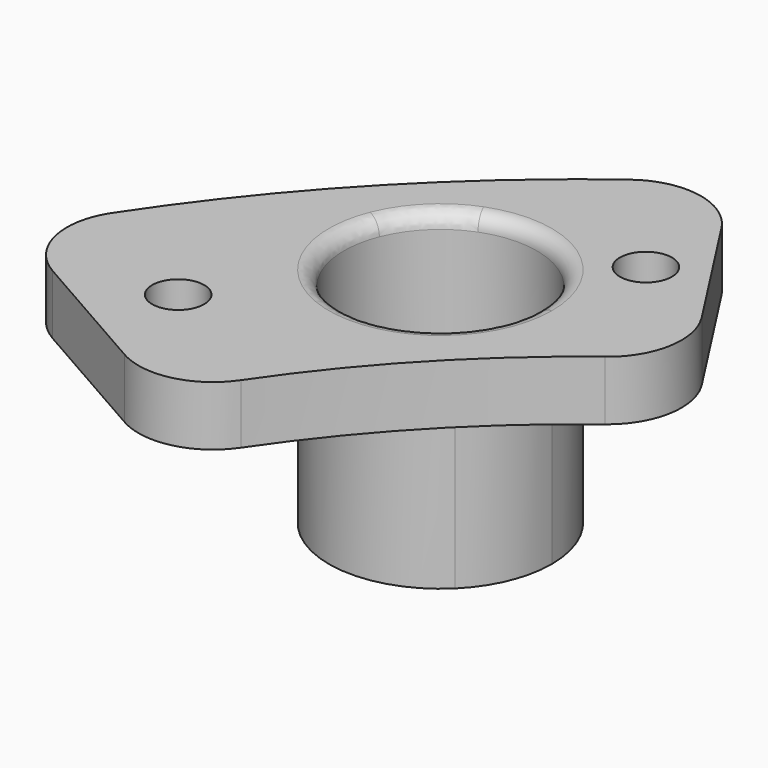
from build123d import *

# Parameters (mm, degrees)
F0_R     = 1.75
F1_DEPTH = 4
F2_DEPTH = 15
F3_R     = 5
F4_R     = 1


# Not quite as in the source:
# - a feature names something its author has since deleted; it is built from what else it names


with BuildPart() as f1:
    # F0 (on Top) → F1 (new body)
    with BuildSketch(Plane.XY):
        with BuildLine():
            Line((-33.9130103109, 52.4991212465), (-41.2382205381, 63.8389314357))
            ThreePointArc((-41.2382205381, 63.8389314357), (-44.9500240756, 61.2820963709), (-48.5037329382, 58.5097247563))
            ThreePointArc((-48.5037329382, 58.5097247563), (-49.20563764, 57.9206804556), (-49.9003894351, 57.3232163633))
            ThreePointArc((-49.9003894351, 57.3232163633), (-44.1059919264, 55.4322284704), (-41.6292667465, 49.8629637))
            ThreePointArc((-41.6292667465, 49.8629637), (-42.2108537269, 46.9671803363), (-43.8654164238, 44.5205036131))
            ThreePointArc((-43.8654164238, 44.5205036131), (-39.0932922784, 48.7643773551), (-33.9130103109, 52.4991212465))
        make_face()
        with Locations((-40.8724684836, 56.828173647)):
            Circle(F0_R, mode=Mode.SUBTRACT)
        with BuildLine():
            ThreePointArc((-49.4610434567, 59.6645219554), (-51.9749220296, 57.4878898553), (-54.3931164452, 55.2054244018))
            ThreePointArc((-54.3931164452, 55.2054244018), (-52.3271541158, 56.6470271117), (-49.9003894351, 57.3232163633))
            ThreePointArc((-49.9003894351, 57.3232163633), (-49.20563764, 57.9206804556), (-48.5037329382, 58.5097247563))
            Line((-48.5037329382, 58.5097247563), (-49.4610434568, 59.6645219554))
        make_face()
        with BuildLine():
            Line((-69.4199358602, 39.5800459158), (-67.3257807989, 38.3860552782))
            ThreePointArc((-67.3257807989, 38.3860552782), (-61.4377349925, 47.2403928751), (-54.3931164452, 55.2054244018))
            ThreePointArc((-54.3931164452, 55.2054244018), (-51.9749220296, 57.4878898553), (-49.4610434567, 59.6645219554))
            Line((-49.4610434568, 59.6645219554), (-50.9995194055, 61.5203750796))
            ThreePointArc((-50.9995194055, 61.5203750796), (-61.2009461738, 51.382406687), (-69.4199358602, 39.5800459158))
        make_face()
        with BuildLine():
            ThreePointArc((-49.4610434567, 59.6645219554), (-45.8371956034, 62.4916114308), (-42.0521327855, 65.0989103456))
            Line((-42.0521327855, 65.0989103456), (-43.360156037, 67.123799043))
            ThreePointArc((-43.360156037, 67.123799043), (-47.2629524833, 64.4354006125), (-50.9995194055, 61.5203750796))
            Line((-50.9995194055, 61.5203750796), (-49.4610434568, 59.6645219554))
        make_face()
        with BuildLine():
            Line((-41.2382205381, 63.8389314357), (-42.0521327855, 65.0989103456))
            ThreePointArc((-42.0521327855, 65.0989103456), (-45.8371956034, 62.4916114308), (-49.4610434567, 59.6645219554))
            Line((-49.4610434568, 59.6645219554), (-48.5037329382, 58.5097247563))
            ThreePointArc((-48.5037329382, 58.5097247563), (-44.9500240756, 61.2820963709), (-41.2382205381, 63.8389314357))
        make_face()
        with BuildLine():
            ThreePointArc((-54.3931164452, 55.2054244018), (-61.4377349925, 47.2403928751), (-67.3257807989, 38.3860552782))
            Line((-67.3257807989, 38.3860552782), (-66.0227011705, 37.6430993696))
            ThreePointArc((-66.0227011705, 37.6430993696), (-61.6490099795, 44.4454673566), (-56.577269857, 50.7445813415))
            ThreePointArc((-56.577269857, 50.7445813415), (-55.8651839567, 53.1610569882), (-54.3931164452, 55.2054244018))
        make_face()
        with BuildLine():
            ThreePointArc((-49.9003894351, 57.3232163633), (-52.3271541158, 56.6470271117), (-54.3931164452, 55.2054244018))
            ThreePointArc((-54.3931164452, 55.2054244018), (-55.8651839567, 53.1610569882), (-56.577269857, 50.7445813415))
            ThreePointArc((-56.577269857, 50.7445813415), (-55.8760464089, 51.5157008854), (-55.1643138946, 52.277131449))
            ThreePointArc((-55.1643138946, 52.277131449), (-53.6912700872, 54.4930960436), (-51.453714731, 55.9331318663))
            ThreePointArc((-51.453714731, 55.9331318663), (-50.6818181556, 56.6334998781), (-49.9003894351, 57.3232163633))
        make_face()
        with BuildLine():
            ThreePointArc((-41.6292667465, 49.8629637), (-44.1059919264, 55.4322284704), (-49.9003894351, 57.3232163633))
            ThreePointArc((-49.9003894351, 57.3232163633), (-50.6818181556, 56.6334998781), (-51.453714731, 55.9331318663))
            ThreePointArc((-51.453714731, 55.9331318663), (-45.4454448113, 55.2182840406), (-42.6292667465, 49.8629637))
            ThreePointArc((-42.6292667465, 49.8629637), (-50.3585335071, 43.4802602578), (-55.1643138946, 52.277131449))
            ThreePointArc((-55.1643138946, 52.277131449), (-55.8760464089, 51.5157008854), (-56.577269857, 50.7445813415))
            ThreePointArc((-56.577269857, 50.7445813415), (-52.4273596413, 43.1270462972), (-43.8654164238, 44.5205036131))
            ThreePointArc((-43.8654164238, 44.5205036131), (-42.2108537269, 46.9671803363), (-41.6292667465, 49.8629637))
        make_face()
        with BuildLine():
            ThreePointArc((-56.577269857, 50.7445813415), (-61.6490099795, 44.4454673566), (-66.0227011705, 37.6430993696))
            Line((-66.0227011705, 37.6430993696), (-54.2949845152, 30.9564961921))
            ThreePointArc((-54.2949845152, 30.9564961921), (-49.5465604503, 38.0970910641), (-43.8654164238, 44.5205036131))
            ThreePointArc((-43.8654164238, 44.5205036131), (-52.4273596413, 43.1270462972), (-56.577269857, 50.7445813415))
        make_face()
        with Locations((-58.1049998349, 39.0359961341)):
            Circle(F0_R, mode=Mode.SUBTRACT)
        with BuildLine():
            ThreePointArc((-43.8654164238, 44.5205036131), (-49.5465604503, 38.0970910641), (-54.2949845152, 30.9564961921))
            Line((-54.2949845152, 30.9564961921), (-51.8884792508, 29.5844178737))
            ThreePointArc((-51.8884792508, 29.5844178737), (-43.387995367, 41.0503826769), (-32.4098910344, 50.1722136548))
            Line((-32.4098910344, 50.1722136548), (-33.9130103109, 52.4991212465))
            ThreePointArc((-33.9130103109, 52.4991212465), (-39.0932922784, 48.7643773551), (-43.8654164238, 44.5205036131))
        make_face()
    extrude(amount=-F1_DEPTH)

    # F0 (on Top) → F2 (join)
    with BuildSketch(Plane.XY):
        with BuildLine():
            ThreePointArc((-49.9003894351, 57.3232163633), (-52.3271541158, 56.6470271117), (-54.3931164452, 55.2054244018))
            ThreePointArc((-54.3931164452, 55.2054244018), (-55.8651839567, 53.1610569882), (-56.577269857, 50.7445813415))
            ThreePointArc((-56.577269857, 50.7445813415), (-55.8760464089, 51.5157008854), (-55.1643138946, 52.277131449))
            ThreePointArc((-55.1643138946, 52.277131449), (-53.6912700872, 54.4930960436), (-51.453714731, 55.9331318663))
            ThreePointArc((-51.453714731, 55.9331318663), (-50.6818181556, 56.6334998781), (-49.9003894351, 57.3232163633))
        make_face()
        with BuildLine():
            ThreePointArc((-41.6292667465, 49.8629637), (-44.1059919264, 55.4322284704), (-49.9003894351, 57.3232163633))
            ThreePointArc((-49.9003894351, 57.3232163633), (-50.6818181556, 56.6334998781), (-51.453714731, 55.9331318663))
            ThreePointArc((-51.453714731, 55.9331318663), (-45.4454448113, 55.2182840406), (-42.6292667465, 49.8629637))
            ThreePointArc((-42.6292667465, 49.8629637), (-50.3585335071, 43.4802602578), (-55.1643138946, 52.277131449))
            ThreePointArc((-55.1643138946, 52.277131449), (-55.8760464089, 51.5157008854), (-56.577269857, 50.7445813415))
            ThreePointArc((-56.577269857, 50.7445813415), (-52.4273596413, 43.1270462972), (-43.8654164238, 44.5205036131))
            ThreePointArc((-43.8654164238, 44.5205036131), (-42.2108537269, 46.9671803363), (-41.6292667465, 49.8629637))
        make_face()
    extrude(amount=-F2_DEPTH)

    # F3
    f3_edges = [f1.edges().sort_by_distance(p)[0] for p in [
        (-43.360156, 67.123799, -2),
        (-32.409891, 50.172214, -2),
        (-69.419936, 39.580046, -2),
        (-51.888479, 29.584418, -2),
    ]]
    fillet(f3_edges, radius=F3_R)

    # F4
    f4_edges = [f1.edges().sort_by_distance(p)[0] for p in [
        (-43.865417, 44.520503, -4),
        (-46.804819, 43.792796, 0),
    ]]
    fillet(f4_edges, radius=F4_R)


solid = f1.part
